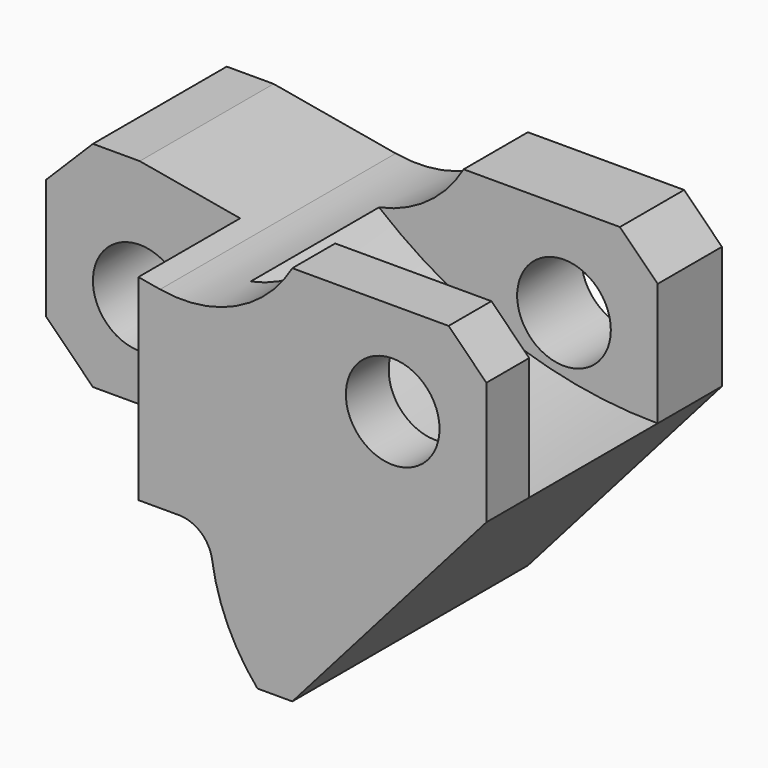
from build123d import *

# Parameters (mm, degrees)
F0_R        = 7
F1_DEPTH    = 22
F3_DEPTH    = 69.1
F4_T4_DEPTH = 24
F2_W        = 40.4194121808
F2_H        = 21.5930561535
F5_DEPTH    = 72.2


# Not quite as in the source:
# - a fillet or chamfer that OpenCascade refuses, or shapes differently, is made with other operations: its cross-section is extruded or revolved along the edge and cut away or added


with BuildPart() as f1:
    # F0 (on Front) → F1 (new body, symmetric)
    with BuildSketch(Plane.XZ):
        with BuildLine():
            Line((-7, 18), (-14, 11))
            Line((-14, 11), (-14, -7))
            Line((-14, -7), (-7, -14))
            Line((-7, -14), (21.0666262554, -14))
            ThreePointArc((21.0666262554, -14), (24.3318620364, -15.2134137678), (26.0122649968, -18.2647058824))
            ThreePointArc((26.0122649968, -18.2647058824), (28.3490951999, -26.115672061), (32.7880673968, -33))
            Line((32.7880673968, -33), (38, -33))
            Line((38, -33), (67, 0))
            Line((67, 0), (67, 18.3546076061))
            Line((67, 18.3546076061), (61.3546076061, 24))
            Line((61.3546076061, 24), (38, 24))
            ThreePointArc((38, 24), (29.5749729609, 16.2760691513), (18.2430849879, 14.7832519053))
            Line((18.2430849879, 14.7832519053), (0, 18))
            Line((0, 18), (-7, 18))
        make_face()
        Circle(F0_R, mode=Mode.SUBTRACT)
        with Locations((53, 10)):
            Circle(F0_R, mode=Mode.SUBTRACT)
    extrude(amount=F1_DEPTH, both=True)

    # F2 (on Top) → F3 (cut)
    with BuildSketch(Plane.XY):
        Polygon((90.3841100792, -14), (90.3841100792, 10), (25.3584354958, 10), (25.3584354958, -14), (86.1629769206, -14), align=None)
    extrude(amount=F3_DEPTH, mode=Mode.SUBTRACT)

    # F4: fillet of radius 65.7 on 1 edges, made by hand


with BuildPart() as f4_tool2:
    # F4_s3 → F4_t4 (new body)
    with BuildSketch(Plane.XZ.offset(-10)):
        with BuildLine():
            ThreePointArc((67, 0), (44.8895413168, 3.8321555148), (25.3584354958, 14.88175752))
            Line((25.3584354958, 14.88175752), (24.5256098882, 13.8653926704))
            ThreePointArc((24.5256098882, 13.8653926704), (24.0444354958, 7.44087876), (24.0444354958, 0))
            Line((24.0444354958, 0), (25.3584354958, -1.314))
            Line((25.3584354958, -1.314), (67.0000056826, -1.314))
            Line((67.0000056826, -1.314), (67, 0))
        make_face()
    extrude(amount=F4_T4_DEPTH)

    split(bisect_by=Plane(origin=(37.8046632124, 0, -33.2222797927), x_dir=(0, 1, 0), z_dir=(-0.7511648984, 0, 0.6601146077)), keep=Keep.TOP)


with BuildPart() as f1_1:
    add(f1.part)

    # F4_t1: union F4_tool2
    add(f4_tool2.part)

    # F2 (on Top) → F5 (cut, symmetric)
    with BuildSketch(Plane.XY):
        with Locations((-5.2097060904, -13.7965280768)):
            Rectangle(F2_W, F2_H)
    extrude(amount=F5_DEPTH, both=True, mode=Mode.SUBTRACT)


solid = f1_1.part
